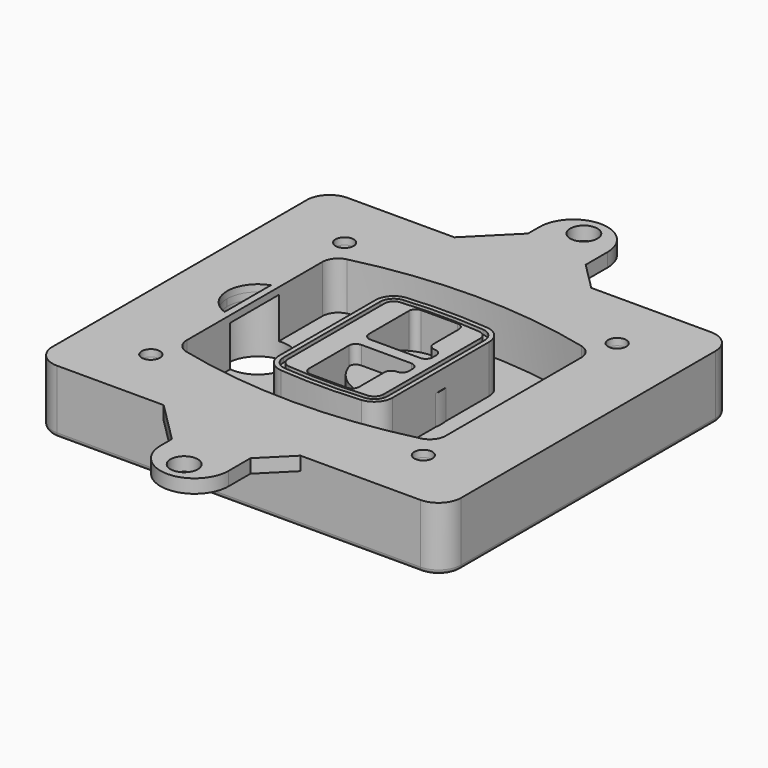
from build123d import *

# Parameters (mm, degrees)
F0_R      = 4
F1_DEPTH  = 25
F2_DEPTH  = 3
F3_DEPTH  = 18
F5_DEPTH  = 21
F6_DEPTH  = 2
F8_DEPTH  = 20
F9_DEPTH  = 16
F10_DEPTH = 25
F7_R      = 6
F7_R_2    = 4
F11_DEPTH = 6
F13_DEPTH = 9
F15_R     = 2
F16_R     = 6
F16_R_2   = 4
F17_DEPTH = 3


# Not quite as in the source:
# - a feature of the source that left no trace in its solid (it failed there, or was rolled back) is left out
# - a feature names something its author has since deleted; it is built from what else it names


with BuildPart() as f1:
    # F0 (on Top) → F1 (new body)
    with BuildSketch(Plane.XY):
        with BuildLine():
            ThreePointArc((-90, -70), (-87.0710678119, -77.0710678119), (-80, -80))
            Line((-80, -80), (80, -80))
            ThreePointArc((80, -80), (87.0710678119, -77.0710678119), (90, -70))
            Line((90, -70), (90, 70))
            ThreePointArc((90, 70), (87.0710678119, 77.0710678119), (80, 80))
            Line((80, 80), (-80, 80))
            ThreePointArc((-80, 80), (-87.0710678119, 77.0710678119), (-90, 70))
            Line((-90, 70), (-90, -70))
        make_face()
        with Locations((-60, -53.3333333333)):
            Circle(F0_R, mode=Mode.SUBTRACT)
        with Locations((60, -53.3333333333)):
            Circle(F0_R, mode=Mode.SUBTRACT)
        with Locations((-60, 53.3333333333)):
            Circle(F0_R, mode=Mode.SUBTRACT)
        with BuildLine():
            ThreePointArc((-64, 37.2990447398), (-61.0143011354, 45.9411029726), (-53.3306899286, 50.8970778549))
            ThreePointArc((-53.3306899286, 50.8970778549), (0, 57.3333333333), (53.3306899286, 50.8970778549))
            ThreePointArc((53.3306899286, 50.8970778549), (61.0143011354, 45.9411029726), (64, 37.2990447398))
            Line((64, 37.2990447398), (64, -37.2990447398))
            ThreePointArc((64, -37.2990447398), (61.0143011354, -45.9411029726), (53.3306899286, -50.8970778549))
            ThreePointArc((53.3306899286, -50.8970778549), (0, -57.3333333333), (-53.3306899286, -50.8970778549))
            ThreePointArc((-53.3306899286, -50.8970778549), (-61.0143011354, -45.9411029726), (-64, -37.2990447398))
            Line((-64, -37.2990447398), (-64, 37.2990447398))
        make_face(mode=Mode.SUBTRACT)
        with Locations((60, 53.3333333333)):
            Circle(F0_R, mode=Mode.SUBTRACT)
        with BuildLine():
            ThreePointArc((53.3306899286, 50.8970778549), (0, 57.3333333333), (-53.3306899286, 50.8970778549))
            ThreePointArc((-53.3306899286, 50.8970778549), (-61.0143011354, 45.9411029726), (-64, 37.2990447398))
            Line((-64, 37.2990447398), (-64, -37.2990447398))
            ThreePointArc((-64, -37.2990447398), (-61.0143011354, -45.9411029726), (-53.3306899286, -50.8970778549))
            ThreePointArc((-53.3306899286, -50.8970778549), (0, -57.3333333333), (53.3306899286, -50.8970778549))
            ThreePointArc((53.3306899286, -50.8970778549), (61.0143011354, -45.9411029726), (64, -37.2990447398))
            Line((64, -37.2990447398), (64, 37.2990447398))
            ThreePointArc((64, 37.2990447398), (61.0143011354, 45.9411029726), (53.3306899286, 50.8970778549))
        make_face()
        with BuildLine():
            Line((-60, -37.2990447398), (-60, 37.2990447398))
            ThreePointArc((-60, 37.2990447398), (-57.8673579538, 43.4719434775), (-52.3790642347, 47.0119255363))
            ThreePointArc((-52.3790642347, 47.0119255363), (0, 53.3333333333), (52.3790642347, 47.0119255363))
            ThreePointArc((52.3790642347, 47.0119255363), (57.8673579538, 43.4719434775), (60, 37.2990447398))
            Line((60, 37.2990447398), (60, -37.2990447398))
            ThreePointArc((60, -37.2990447398), (57.8673579538, -43.4719434775), (52.3790642347, -47.0119255363))
            ThreePointArc((52.3790642347, -47.0119255363), (0, -53.3333333333), (-52.3790642347, -47.0119255363))
            ThreePointArc((-52.3790642347, -47.0119255363), (-57.8673579538, -43.4719434775), (-60, -37.2990447398))
        make_face(mode=Mode.SUBTRACT)
        with BuildLine():
            ThreePointArc((-52.3790642347, 47.0119255363), (-57.8673579538, 43.4719434775), (-60, 37.2990447398))
            Line((-60, 37.2990447398), (-60, -37.2990447398))
            ThreePointArc((-60, -37.2990447398), (-57.8673579538, -43.4719434775), (-52.3790642347, -47.0119255363))
            ThreePointArc((-52.3790642347, -47.0119255363), (0, -53.3333333333), (52.3790642347, -47.0119255363))
            ThreePointArc((52.3790642347, -47.0119255363), (57.8673579538, -43.4719434775), (60, -37.2990447398))
            Line((60, -37.2990447398), (60, 37.2990447398))
            ThreePointArc((60, 37.2990447398), (57.8673579538, 43.4719434775), (52.3790642347, 47.0119255363))
            ThreePointArc((52.3790642347, 47.0119255363), (0, 53.3333333333), (-52.3790642347, 47.0119255363))
        make_face()
        with BuildLine():
            ThreePointArc((51.6653449643, 44.0980612973), (55.5071505677, 41.6200738562), (57, 37.2990447398))
            Line((57, 37.2990447398), (57, -37.2990447398))
            ThreePointArc((57, -37.2990447398), (55.5071505677, -41.6200738562), (51.6653449643, -44.0980612973))
            ThreePointArc((51.6653449643, -44.0980612973), (0, -50.3333333333), (-51.6653449643, -44.0980612973))
            ThreePointArc((-51.6653449643, -44.0980612973), (-55.5071505677, -41.6200738562), (-57, -37.2990447398))
            Line((-57, -37.2990447398), (-57, 37.2990447398))
            ThreePointArc((-57, 37.2990447398), (-55.5071505677, 41.6200738562), (-51.6653449643, 44.0980612973))
            ThreePointArc((-51.6653449643, 44.0980612973), (0, 50.3333333333), (51.6653449643, 44.0980612973))
        make_face(mode=Mode.SUBTRACT)
        with BuildLine():
            Line((57, -37.2990447398), (57, 37.2990447398))
            ThreePointArc((57, 37.2990447398), (55.5071505677, 41.6200738562), (51.6653449643, 44.0980612973))
            ThreePointArc((51.6653449643, 44.0980612973), (0, 50.3333333333), (-51.6653449643, 44.0980612973))
            ThreePointArc((-51.6653449643, 44.0980612973), (-55.5071505677, 41.6200738562), (-57, 37.2990447398))
            Line((-57, 37.2990447398), (-57, -37.2990447398))
            ThreePointArc((-57, -37.2990447398), (-55.5071505677, -41.6200738562), (-51.6653449643, -44.0980612973))
            ThreePointArc((-51.6653449643, -44.0980612973), (0, -50.3333333333), (51.6653449643, -44.0980612973))
            ThreePointArc((51.6653449643, -44.0980612973), (55.5071505677, -41.6200738562), (57, -37.2990447398))
        make_face()
    extrude(amount=-F1_DEPTH)

    # F0 (on Top) → F2 (join)
    with BuildSketch(Plane.XY):
        with BuildLine():
            ThreePointArc((-52.3790642347, 47.0119255363), (-57.8673579538, 43.4719434775), (-60, 37.2990447398))
            Line((-60, 37.2990447398), (-60, -37.2990447398))
            ThreePointArc((-60, -37.2990447398), (-57.8673579538, -43.4719434775), (-52.3790642347, -47.0119255363))
            ThreePointArc((-52.3790642347, -47.0119255363), (0, -53.3333333333), (52.3790642347, -47.0119255363))
            ThreePointArc((52.3790642347, -47.0119255363), (57.8673579538, -43.4719434775), (60, -37.2990447398))
            Line((60, -37.2990447398), (60, 37.2990447398))
            ThreePointArc((60, 37.2990447398), (57.8673579538, 43.4719434775), (52.3790642347, 47.0119255363))
            ThreePointArc((52.3790642347, 47.0119255363), (0, 53.3333333333), (-52.3790642347, 47.0119255363))
        make_face()
        with BuildLine():
            ThreePointArc((51.6653449643, 44.0980612973), (55.5071505677, 41.6200738562), (57, 37.2990447398))
            Line((57, 37.2990447398), (57, -37.2990447398))
            ThreePointArc((57, -37.2990447398), (55.5071505677, -41.6200738562), (51.6653449643, -44.0980612973))
            ThreePointArc((51.6653449643, -44.0980612973), (0, -50.3333333333), (-51.6653449643, -44.0980612973))
            ThreePointArc((-51.6653449643, -44.0980612973), (-55.5071505677, -41.6200738562), (-57, -37.2990447398))
            Line((-57, -37.2990447398), (-57, 37.2990447398))
            ThreePointArc((-57, 37.2990447398), (-55.5071505677, 41.6200738562), (-51.6653449643, 44.0980612973))
            ThreePointArc((-51.6653449643, 44.0980612973), (0, 50.3333333333), (51.6653449643, 44.0980612973))
        make_face(mode=Mode.SUBTRACT)
    extrude(amount=F2_DEPTH)

    # F0 (on Top) → F3 (cut)
    with BuildSketch(Plane.XY):
        with BuildLine():
            Line((57, -37.2990447398), (57, 37.2990447398))
            ThreePointArc((57, 37.2990447398), (55.5071505677, 41.6200738562), (51.6653449643, 44.0980612973))
            ThreePointArc((51.6653449643, 44.0980612973), (0, 50.3333333333), (-51.6653449643, 44.0980612973))
            ThreePointArc((-51.6653449643, 44.0980612973), (-55.5071505677, 41.6200738562), (-57, 37.2990447398))
            Line((-57, 37.2990447398), (-57, -37.2990447398))
            ThreePointArc((-57, -37.2990447398), (-55.5071505677, -41.6200738562), (-51.6653449643, -44.0980612973))
            ThreePointArc((-51.6653449643, -44.0980612973), (0, -50.3333333333), (51.6653449643, -44.0980612973))
            ThreePointArc((51.6653449643, -44.0980612973), (55.5071505677, -41.6200738562), (57, -37.2990447398))
        make_face()
    extrude(amount=-F3_DEPTH, mode=Mode.SUBTRACT)

    # F4 (on face) → F5 (join, through all)
    with BuildSketch(Plane.XY.offset(3)):
        with BuildLine():
            ThreePointArc((-25, -26.587695628), (-22.8992979869, -31.9912392117), (-17.7004291845, -34.5569740744))
            ThreePointArc((-17.7004291845, -34.5569740744), (0, -35.3333333333), (17.7004291845, -34.5569740744))
            ThreePointArc((17.7004291845, -34.5569740744), (22.8992979869, -31.9912392117), (25, -26.587695628))
            Line((25, -26.587695628), (25, 26.587695628))
            ThreePointArc((25, 26.587695628), (22.8992979869, 31.9912392117), (17.7004291845, 34.5569740744))
            ThreePointArc((17.7004291845, 34.5569740744), (0, 35.3333333333), (-17.7004291845, 34.5569740744))
            ThreePointArc((-17.7004291845, 34.5569740744), (-22.8992979869, 31.9912392117), (-25, 26.587695628))
            Line((-25, 26.587695628), (-25, -26.587695628))
        make_face()
        with BuildLine():
            ThreePointArc((17.5253218884, 32.5646544628), (21.4244734902, 30.6403533158), (23, 26.587695628))
            Line((23, 26.587695628), (23, -26.587695628))
            ThreePointArc((23, -26.587695628), (21.4244734902, -30.6403533158), (17.5253218884, -32.5646544628))
            ThreePointArc((17.5253218884, -32.5646544628), (0, -33.3333333333), (-17.5253218884, -32.5646544628))
            ThreePointArc((-17.5253218884, -32.5646544628), (-21.4244734902, -30.6403533158), (-23, -26.587695628))
            Line((-23, -26.587695628), (-23, 26.587695628))
            ThreePointArc((-23, 26.587695628), (-21.4244734902, 30.6403533158), (-17.5253218884, 32.5646544628))
            ThreePointArc((-17.5253218884, 32.5646544628), (0, 33.3333333333), (17.5253218884, 32.5646544628))
        make_face(mode=Mode.SUBTRACT)
        with BuildLine():
            Line((23, -26.587695628), (23, 26.587695628))
            ThreePointArc((23, 26.587695628), (21.4244734902, 30.6403533158), (17.5253218884, 32.5646544628))
            ThreePointArc((17.5253218884, 32.5646544628), (0, 33.3333333333), (-17.5253218884, 32.5646544628))
            ThreePointArc((-17.5253218884, 32.5646544628), (-21.4244734902, 30.6403533158), (-23, 26.587695628))
            Line((-23, 26.587695628), (-23, -26.587695628))
            ThreePointArc((-23, -26.587695628), (-21.4244734902, -30.6403533158), (-17.5253218884, -32.5646544628))
            ThreePointArc((-17.5253218884, -32.5646544628), (0, -33.3333333333), (17.5253218884, -32.5646544628))
            ThreePointArc((17.5253218884, -32.5646544628), (21.4244734902, -30.6403533158), (23, -26.587695628))
        make_face()
        with BuildLine():
            ThreePointArc((17.3502145923, 30.5723348512), (19.9496489934, 29.2894674198), (21, 26.587695628))
            Line((21, 26.587695628), (21, -26.587695628))
            ThreePointArc((21, -26.587695628), (19.9496489934, -29.2894674198), (17.3502145923, -30.5723348512))
            ThreePointArc((17.3502145923, -30.5723348512), (0, -31.3333333333), (-17.3502145923, -30.5723348512))
            ThreePointArc((-17.3502145923, -30.5723348512), (-19.9496489934, -29.2894674198), (-21, -26.587695628))
            Line((-21, -26.587695628), (-21, 26.587695628))
            ThreePointArc((-21, 26.587695628), (-19.9496489934, 29.2894674198), (-17.3502145923, 30.5723348512))
            ThreePointArc((-17.3502145923, 30.5723348512), (0, 31.3333333333), (17.3502145923, 30.5723348512))
        make_face(mode=Mode.SUBTRACT)
        with BuildLine():
            Line((21, -26.587695628), (21, 26.587695628))
            ThreePointArc((21, 26.587695628), (19.9496489934, 29.2894674198), (17.3502145923, 30.5723348512))
            ThreePointArc((17.3502145923, 30.5723348512), (0, 31.3333333333), (-17.3502145923, 30.5723348512))
            ThreePointArc((-17.3502145923, 30.5723348512), (-19.9496489934, 29.2894674198), (-21, 26.587695628))
            Line((-21, 26.587695628), (-21, -26.587695628))
            ThreePointArc((-21, -26.587695628), (-19.9496489934, -29.2894674198), (-17.3502145923, -30.5723348512))
            ThreePointArc((-17.3502145923, -30.5723348512), (0, -31.3333333333), (17.3502145923, -30.5723348512))
            ThreePointArc((17.3502145923, -30.5723348512), (19.9496489934, -29.2894674198), (21, -26.587695628))
        make_face()
        with BuildLine():
            Line((-8, -2.5), (14, -2.5))
            ThreePointArc((14, -2.5), (16.1213203436, -3.3786796564), (17, -5.5))
            Line((17, -5.5), (17, -7.5))
            ThreePointArc((17, -7.5), (16.1213203436, -9.6213203436), (14, -10.5))
            ThreePointArc((14, -10.5), (11.8786796564, -11.3786796564), (11, -13.5))
            Line((11, -13.5), (11, -27.5))
            ThreePointArc((11, -27.5), (10.1213203436, -29.6213203436), (8, -30.5))
            Line((8, -30.5), (-8, -30.5))
            ThreePointArc((-8, -30.5), (-10.1213203436, -29.6213203436), (-11, -27.5))
            Line((-11, -27.5), (-11, -5.5))
            ThreePointArc((-11, -5.5), (-10.1213203436, -3.3786796564), (-8, -2.5))
        make_face(mode=Mode.SUBTRACT)
        with BuildLine():
            ThreePointArc((-8, 2.5), (-10.1213203436, 3.3786796564), (-11, 5.5))
            Line((-11, 5.5), (-11, 27.5))
            ThreePointArc((-11, 27.5), (-10.1213203436, 29.6213203436), (-8, 30.5))
            Line((-8, 30.5), (8, 30.5))
            ThreePointArc((8, 30.5), (10.1213203436, 29.6213203436), (11, 27.5))
            Line((11, 27.5), (11, 13.5))
            ThreePointArc((11, 13.5), (11.8786796564, 11.3786796564), (14, 10.5))
            ThreePointArc((14, 10.5), (16.1213203436, 9.6213203436), (17, 7.5))
            Line((17, 7.5), (17, 5.5))
            ThreePointArc((17, 5.5), (16.1213203436, 3.3786796564), (14, 2.5))
            Line((14, 2.5), (-8, 2.5))
        make_face(mode=Mode.SUBTRACT)
    extrude(amount=-F5_DEPTH)

    # F4 (on face) → F6 (cut)
    with BuildSketch(Plane.XY.offset(3)):
        with BuildLine():
            Line((23, -26.587695628), (23, 26.587695628))
            ThreePointArc((23, 26.587695628), (21.4244734902, 30.6403533158), (17.5253218884, 32.5646544628))
            ThreePointArc((17.5253218884, 32.5646544628), (0, 33.3333333333), (-17.5253218884, 32.5646544628))
            ThreePointArc((-17.5253218884, 32.5646544628), (-21.4244734902, 30.6403533158), (-23, 26.587695628))
            Line((-23, 26.587695628), (-23, -26.587695628))
            ThreePointArc((-23, -26.587695628), (-21.4244734902, -30.6403533158), (-17.5253218884, -32.5646544628))
            ThreePointArc((-17.5253218884, -32.5646544628), (0, -33.3333333333), (17.5253218884, -32.5646544628))
            ThreePointArc((17.5253218884, -32.5646544628), (21.4244734902, -30.6403533158), (23, -26.587695628))
        make_face()
        with BuildLine():
            ThreePointArc((17.3502145923, 30.5723348512), (19.9496489934, 29.2894674198), (21, 26.587695628))
            Line((21, 26.587695628), (21, -26.587695628))
            ThreePointArc((21, -26.587695628), (19.9496489934, -29.2894674198), (17.3502145923, -30.5723348512))
            ThreePointArc((17.3502145923, -30.5723348512), (0, -31.3333333333), (-17.3502145923, -30.5723348512))
            ThreePointArc((-17.3502145923, -30.5723348512), (-19.9496489934, -29.2894674198), (-21, -26.587695628))
            Line((-21, -26.587695628), (-21, 26.587695628))
            ThreePointArc((-21, 26.587695628), (-19.9496489934, 29.2894674198), (-17.3502145923, 30.5723348512))
            ThreePointArc((-17.3502145923, 30.5723348512), (0, 31.3333333333), (17.3502145923, 30.5723348512))
        make_face(mode=Mode.SUBTRACT)
    extrude(amount=-F6_DEPTH, mode=Mode.SUBTRACT)

    # F7 (on face) → F8 (join)
    with BuildSketch(Plane(origin=(0, 0, -25), x_dir=(1, 0, 0), z_dir=(0, 0, -1))):
        with BuildLine():
            ThreePointArc((-6.71157564, 0), (6.7567035675, 13.4682792075), (20.224982775, 0))
            Line((20.224982775, 0), (25.224982775, 0))
            ThreePointArc((25.224982775, 0), (6.7567035675, 18.4682792075), (-11.71157564, 0))
            Line((-11.71157564, 0), (-6.71157564, 0))
        make_face()
        with BuildLine():
            Line((-6.71157564, 0), (20.224982775, 0))
            ThreePointArc((20.224982775, 0), (6.7567035675, 13.4682792075), (-6.71157564, 0))
        make_face()
        with BuildLine():
            ThreePointArc((-6.71157564, 0), (6.7567035675, -13.4682792075), (20.224982775, 0))
            Line((20.224982775, 0), (-6.71157564, 0))
        make_face()
        with BuildLine():
            Line((25.224982775, 0), (20.224982775, 0))
            ThreePointArc((20.224982775, 0), (6.7567035675, -13.4682792075), (-6.71157564, 0))
            Line((-6.71157564, 0), (-11.71157564, 0))
            ThreePointArc((-11.71157564, 0), (6.7567035675, -18.4682792075), (25.224982775, 0))
        make_face()
    extrude(amount=-F8_DEPTH)

    # F7 (on face) → F9 (cut)
    with BuildSketch(Plane(origin=(0, 0, -25), x_dir=(1, 0, 0), z_dir=(0, 0, -1))):
        with BuildLine():
            Line((-6.71157564, 0), (20.224982775, 0))
            ThreePointArc((20.224982775, 0), (6.7567035675, 13.4682792075), (-6.71157564, 0))
        make_face()
        with BuildLine():
            ThreePointArc((-6.71157564, 0), (6.7567035675, -13.4682792075), (20.224982775, 0))
            Line((20.224982775, 0), (-6.71157564, 0))
        make_face()
    extrude(amount=-F9_DEPTH, mode=Mode.SUBTRACT)

    # F7 (on face) → F10 (cut)
    with BuildSketch(Plane(origin=(0, 0, -25), x_dir=(1, 0, 0), z_dir=(0, 0, -1))):
        with BuildLine():
            Line((-69.0318229325, 0), (-42.0952645175, 0))
            ThreePointArc((-42.0952645175, 0), (-55.563543725, 13.4682792075), (-69.0318229325, 0))
        make_face()
        with BuildLine():
            ThreePointArc((-69.0318229325, 0), (-55.563543725, -13.4682792075), (-42.0952645175, 0))
            Line((-42.0952645175, 0), (-69.0318229325, 0))
        make_face()
    extrude(amount=-F10_DEPTH, mode=Mode.SUBTRACT)

    # F7 (on face) → F11 (cut)
    with BuildSketch(Plane(origin=(0, 0, -25), x_dir=(1, 0, 0), z_dir=(0, 0, -1))):
        with Locations((60, -53.3333333333)):
            Circle(F7_R)
        with Locations((60, -53.3333333333)):
            Circle(F7_R_2, mode=Mode.SUBTRACT)
        with Locations((-60, -53.3333333333)):
            Circle(F7_R)
        with Locations((-60, -53.3333333333)):
            Circle(F7_R_2, mode=Mode.SUBTRACT)
        with Locations((-60, 53.3333333333)):
            Circle(F7_R)
        with Locations((-60, 53.3333333333)):
            Circle(F7_R_2, mode=Mode.SUBTRACT)
        with Locations((60, 53.3333333333)):
            Circle(F7_R)
        with Locations((60, 53.3333333333)):
            Circle(F7_R_2, mode=Mode.SUBTRACT)
    extrude(amount=-F11_DEPTH, mode=Mode.SUBTRACT)

    # F12 (on face) → F13 (cut, through all)
    with BuildSketch(Plane(origin=(0, 0, -9), x_dir=(1, 0, 0), z_dir=(0, 0, -1))):
        with BuildLine():
            ThreePointArc((20.224982775, 0), (20.1663399806, 1.2554664788), (19.9909222755, 2.5))
            Line((19.9909222755, 2.5), (14, 2.5))
            ThreePointArc((14, 2.5), (16.1213203436, 3.3786796564), (17, 5.5))
            Line((17, 5.5), (17, 7.5))
            ThreePointArc((17, 7.5), (16.1213203436, 9.6213203436), (14, 10.5))
            ThreePointArc((14, 10.5), (12.1627255951, 11.1284134507), (11.0951631559, 12.750384826))
            ThreePointArc((11.0951631559, 12.750384826), (11.0476113807, 12.7664660322), (11, 12.7823698976))
            Line((11, 12.7823698976), (11, -12.7823698976))
            ThreePointArc((11, -12.7823698976), (11.0476113807, -12.7664660322), (11.0951631559, -12.750384826))
            ThreePointArc((11.0951631559, -12.750384826), (12.1627255951, -11.1284134507), (14, -10.5))
            ThreePointArc((14, -10.5), (16.1213203436, -9.6213203436), (17, -7.5))
            Line((17, -7.5), (17, -5.5))
            ThreePointArc((17, -5.5), (16.1213203436, -3.3786796564), (14, -2.5))
            Line((14, -2.5), (19.9909222755, -2.5))
            ThreePointArc((19.9909222755, -2.5), (20.1663399806, -1.2554664788), (20.224982775, 0))
        make_face()
    extrude(amount=F13_DEPTH, mode=Mode.SUBTRACT)

    # F15
    f15_edges = [f1.edges().sort_by_distance(p)[0] for p in [
        (0, -80, -25),
        (-87.071068, -77.071068, -25),
        (-90, 0, -25),
        (-87.071068, 77.071068, -25),
        (87.071068, -77.071068, -25),
        (0, 80, -25),
        (90, 0, -25),
        (87.071068, 77.071068, -25),
    ]]
    fillet(f15_edges, radius=F15_R)

    # F16 (on face) → F17 (join, symmetric)
    with BuildSketch(Plane.XY):
        with BuildLine():
            Line((-15, 98), (-33, 80))
            Line((-33, 80), (27.25, 80))
            Line((27.25, 80), (15, 92.25))
            Line((15, 92.25), (15, 104.25))
            ThreePointArc((15, 104.25), (0, 119.25), (-15, 104.25))
            Line((-15, 104.25), (-15, 98))
        make_face()
        with Locations((0, 110)):
            Circle(F16_R, mode=Mode.SUBTRACT)
        with BuildLine():
            Line((-33, 80), (-80, 80))
            ThreePointArc((-80, 80), (-87.0710678119, 77.0710678119), (-90, 70))
            Line((-90, 70), (-90, -70))
            ThreePointArc((-90, -70), (-87.0710678119, -77.0710678119), (-80, -80))
            Line((-80, -80), (-33, -80))
            Line((-33, -80), (27.25, -80))
            Line((27.25, -80), (80, -80))
            ThreePointArc((80, -80), (87.0710678119, -77.0710678119), (90, -70))
            Line((90, -70), (90, 70))
            ThreePointArc((90, 70), (87.0710678119, 77.0710678119), (80, 80))
            Line((80, 80), (27.25, 80))
            Line((27.25, 80), (-33, 80))
        make_face()
        with Locations((-60, -53.3333333333)):
            Circle(F16_R_2, mode=Mode.SUBTRACT)
        with Locations((60, -53.3333333333)):
            Circle(F16_R_2, mode=Mode.SUBTRACT)
        with Locations((-60, 53.3333333333)):
            Circle(F16_R_2, mode=Mode.SUBTRACT)
        with BuildLine():
            ThreePointArc((60, -37.2990447398), (57.8673579538, -43.4719434775), (52.3790642347, -47.0119255363))
            ThreePointArc((52.3790642347, -47.0119255363), (0, -53.3333333333), (-52.3790642347, -47.0119255363))
            ThreePointArc((-52.3790642347, -47.0119255363), (-57.8673579538, -43.4719434775), (-60, -37.2990447398))
            Line((-60, -37.2990447398), (-60, -12.7166190685))
            ThreePointArc((-60, -12.7166190685), (-66.5441169481, -7.798817635), (-69.0318229325, 0))
            ThreePointArc((-69.0318229325, 0), (-66.5441169481, 7.798817635), (-60, 12.7166190685))
            Line((-60, 12.7166190685), (-60, 37.2990447398))
            ThreePointArc((-60, 37.2990447398), (-57.8673579538, 43.4719434775), (-52.3790642347, 47.0119255363))
            ThreePointArc((-52.3790642347, 47.0119255363), (0, 53.3333333333), (52.3790642347, 47.0119255363))
            ThreePointArc((52.3790642347, 47.0119255363), (57.8673579538, 43.4719434775), (60, 37.2990447398))
            Line((60, 37.2990447398), (60, -37.2990447398))
        make_face(mode=Mode.SUBTRACT)
        with Locations((60, 53.3333333333)):
            Circle(F16_R_2, mode=Mode.SUBTRACT)
        with BuildLine():
            Line((27.25, -80), (-33, -80))
            Line((-33, -80), (-15, -98))
            Line((-15, -98), (-15, -104.25))
            ThreePointArc((-15, -104.25), (0, -119.25), (15, -104.25))
            Line((15, -104.25), (15, -92.25))
            Line((15, -92.25), (27.25, -80))
        make_face()
        with Locations((0, -110)):
            Circle(F16_R, mode=Mode.SUBTRACT)
    extrude(amount=F17_DEPTH, both=True)


solid = f1.part
